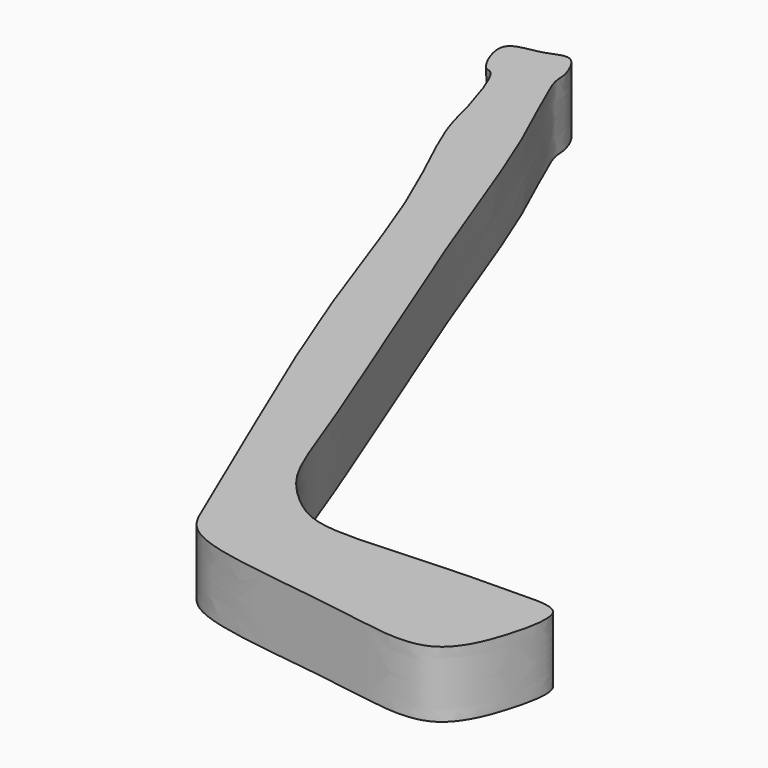
from build123d import *

# Parameters (mm, degrees)
F1_DEPTH = 4


with BuildPart() as f1:
    # F0 (on Top) → F1 (new body)
    with BuildSketch(Plane.XY):
        with BuildLine():
            add(Edge.make_bspline(
                [(-41.8405234814, 41.576500982), (-41.2756549979, 40.050161733), (-38.7554814539, 35.2799722842), (-35.6693893631, 25.7836878676), (-31.4205632812, 15.2640216764), (-26.9574393655, 5.1878876169), (-25.8261755279, 1.9678871554), (-21.7053599167, 0.8585764454), (-14.8958864144, 0.1871575539), (-8.7283496251, -1.2327251094), (-7.163756936, 3.5224157584), (-6.8396922591, 5.2953236731), (-7.0644775675, 6.6653817783), (-9.8466335717, 6.6651361239), (-15.861581921, 6.5241170497), (-21.2885182258, 6.022851137), (-23.5432878903, 7.5080935146), (-25.6416865806, 9.6589473346), (-27.344420002, 14.9640125097), (-34.5328510969, 32.3535899585), (-38.1299849231, 42.8131223834), (-41.1043656621, 48.5394918336), (-40.8789636798, 49.3587895315), (-41.7372767722, 51.4434704176), (-43.2068150975, 50.3887045839), (-45.8103981353, 50.424632306), (-44.4212977902, 47.4327862859), (-43.749191593, 47.7440821239), (-42.4800625696, 44.1540081563), (-42.2228646083, 42.6096304371), (-41.8405234814, 41.576500982)],
                knots=[0, 0, 0, 0, 0.044078894, 0.0988345667, 0.158445142, 0.21493391, 0.2445290992, 0.2777278111, 0.3242289295, 0.3644796163, 0.3990600428, 0.422678219, 0.4397074923, 0.4657598558, 0.5093054427, 0.5491745963, 0.5760942414, 0.6040109182, 0.6438800734, 0.718617168, 0.7789394617, 0.8189588942, 0.8346576216, 0.8568589227, 0.8777795184, 0.9014858675, 0.9274984995, 0.9391906305, 0.9701644286, 1, 1, 1, 1], degree=3))
        make_face()
    extrude(amount=F1_DEPTH)


solid = f1.part
